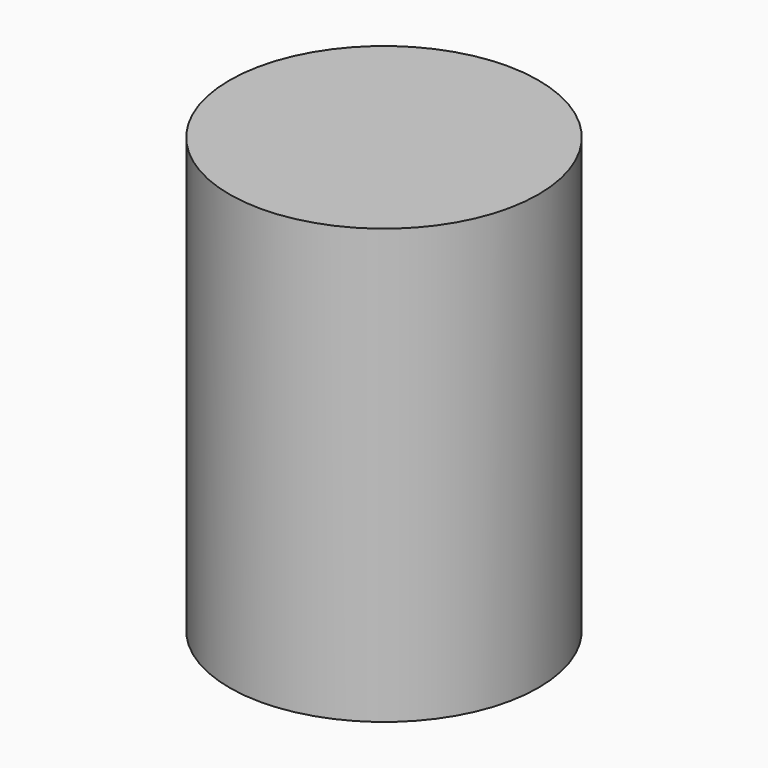
from build123d import *


# Not quite as in the source:
# - a feature of the source that left no trace in its solid (it failed there, or was rolled back) is left out


with BuildPart() as f1:
    # F0 (on Right) → F1 (revolve)
    with BuildSketch(Plane.YZ):
        Polygon((-248.5, 807.6172916793), (-248.5, 149.1172916793), (-248.5, 109.1172916793), (0, 109.1172916793), (0, 807.6172916793), align=None)
    revolve(axis=Axis((0, 0, -107.16170392), (0, 0, -1)))


solid = f1.part
